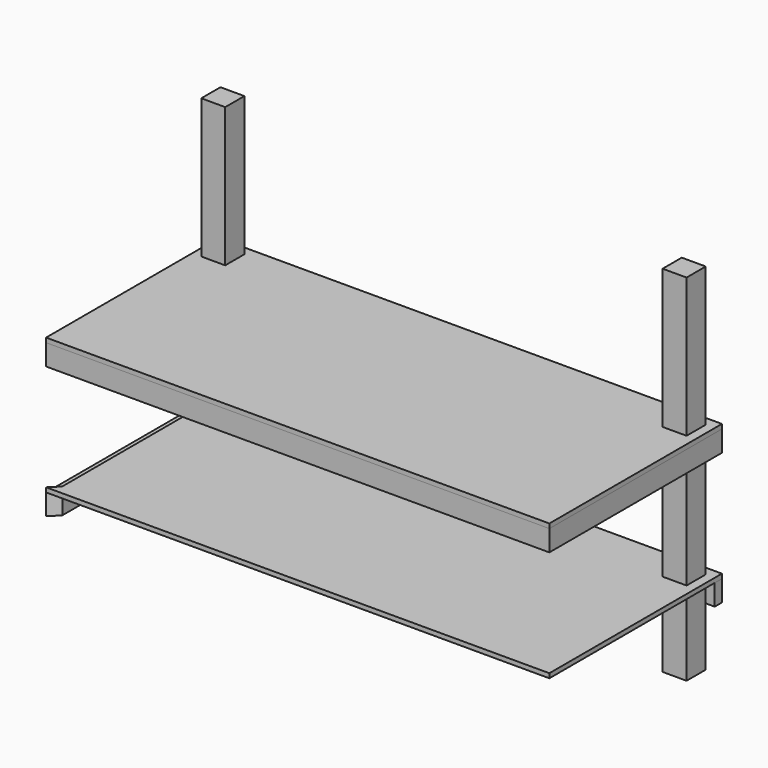
from build123d import *

# Parameters (mm, degrees)
F0_W           = 2133.6
F0_H           = 914.4
F0_W_2         = 101.6
F0_H_2         = 101.6
F1_DEPTH       = 19.05
F2_W           = 2133.6
F2_H           = 88.9
F3_DEPTH       = 38.1
F4_SIZE        = 38.09999
F5_SIZE        = 38.09999
F6_W           = 914.4
F6_H           = 88.9
F7_DEPTH       = 38.1
F8_SIZE        = 38.09999
F9_SIZE        = 38.09999
F10_W          = 2133.6
F10_H          = 88.9
F11_DEPTH      = 38.1
F12_SIZE       = 38.09999
F13_SIZE       = 38.09999
F14_W          = 914.4
F14_H          = 88.9
F15_DEPTH      = 38.1
F16_SIZE       = 38.09999
F17_DEPTH      = 914.4
F17_DEPTH_BACK = 590.55
F18_W          = 914.4
F18_H          = 88.9
F19_DEPTH      = 38.1
F20_SIZE       = 38.09999
F23_DEPTH      = 19.05
F21_W          = 2133.6
F21_H          = 88.9
F24_DEPTH      = 38.1
F25_SIZE       = 38.09999


# Not quite as in the source:
# - a fillet or chamfer is up to 0.001 mm smaller than in the source, because OpenCascade refuses the exact size


with BuildPart() as f1:
    # F0 (on Top) → F1 (new body)
    with BuildSketch(Plane.XY):
        Rectangle(F0_W, F0_H)
        with Locations((-977.9, 368.3)):
            Rectangle(F0_W_2, F0_H_2, mode=Mode.SUBTRACT)
        with Locations((977.9, 368.3)):
            Rectangle(F0_W_2, F0_H_2, mode=Mode.SUBTRACT)
    extrude(amount=-F1_DEPTH)


with BuildPart() as f3:
    # F2 (on face) → F3 (new body)
    with BuildSketch(Plane.XZ.offset(457.2)):
        with Locations((0, -63.5)):
            Rectangle(F2_W, F2_H)
    extrude(amount=-F3_DEPTH)

    # F4 (size 38.1 in the source; OpenCascade refuses exactly that, so slightly less here)
    f4_edges = [f3.edges().sort_by_distance(p)[0] for p in [
        (-1066.8, -419.1, -63.5),
    ]]
    chamfer(f4_edges, length=F4_SIZE)

    # F5 (size 38.1 in the source; OpenCascade refuses exactly that, so slightly less here)
    f5_edges = [f3.edges().sort_by_distance(p)[0] for p in [
        (1066.8, -419.1, -63.5),
    ]]
    chamfer(f5_edges, length=F5_SIZE)


with BuildPart() as f7:
    # F6 (on face) → F7 (new body)
    with BuildSketch(Plane.YZ.offset(1066.8)):
        with Locations((0, -63.5)):
            Rectangle(F6_W, F6_H)
    extrude(amount=-F7_DEPTH)

    # F8 (size 38.1 in the source; OpenCascade refuses exactly that, so slightly less here)
    f8_edges = [f7.edges().sort_by_distance(p)[0] for p in [
        (1028.7, -457.2, -63.5),
    ]]
    chamfer(f8_edges, length=F8_SIZE)

    # F9 (size 38.1 in the source; OpenCascade refuses exactly that, so slightly less here)
    f9_edges = [f7.edges().sort_by_distance(p)[0] for p in [
        (1028.7, 457.2, -63.5),
    ]]
    chamfer(f9_edges, length=F9_SIZE)


with BuildPart() as f11:
    # F10 (on face) → F11 (new body)
    with BuildSketch(Plane(origin=(0, 457.2, 0), x_dir=(-1, 0, 0), z_dir=(0, 1, 0))):
        with Locations((0, -63.5)):
            Rectangle(F10_W, F10_H)
    extrude(amount=-F11_DEPTH)

    # F12 (size 38.1 in the source; OpenCascade refuses exactly that, so slightly less here)
    f12_edges = [f11.edges().sort_by_distance(p)[0] for p in [
        (1066.8, 419.1, -63.5),
    ]]
    chamfer(f12_edges, length=F12_SIZE)

    # F13 (size 38.1 in the source; OpenCascade refuses exactly that, so slightly less here)
    f13_edges = [f11.edges().sort_by_distance(p)[0] for p in [
        (-1066.8, 419.1, -63.5),
    ]]
    chamfer(f13_edges, length=F13_SIZE)


with BuildPart() as f15:
    # F14 (on face) → F15 (new body)
    with BuildSketch(Plane(origin=(-1066.8, 0, 0), x_dir=(0, -1, 0), z_dir=(-1, 0, 0))):
        with Locations((0, -63.5)):
            Rectangle(F14_W, F14_H)
    extrude(amount=-F15_DEPTH)

    # F16 (size 38.1 in the source; OpenCascade refuses exactly that, so slightly less here)
    f16_edges = [f15.edges().sort_by_distance(p)[0] for p in [
        (-1028.7, 457.2, -63.5),
        (-1028.7, -457.2, -63.5),
    ]]
    chamfer(f16_edges, length=F16_SIZE)


with BuildPart() as f17:
    # F0 (on Top) → F17 (new body, two sides)
    with BuildSketch(Plane.XY) as f17_sk:
        with Locations((-977.9, 368.3)):
            Rectangle(F0_W_2, F0_H_2)
    extrude(amount=-F17_DEPTH)
    extrude(f17_sk.sketch, amount=F17_DEPTH_BACK)

    # F18 (on face) → F19 (join)
    with BuildSketch(Plane(origin=(-1066.8, 0, 0), x_dir=(0, -1, 0), z_dir=(-1, 0, 0))):
        with Locations((0, -622.3)):
            Rectangle(F18_W, F18_H)
    extrude(amount=-F19_DEPTH)

    # F20 (size 38.1 in the source; OpenCascade refuses exactly that, so slightly less here)
    f20_edges = [f17.edges().sort_by_distance(p)[0] for p in [
        (-1028.7, -457.2, -622.3),
        (-1028.7, 457.2, -622.3),
    ]]
    chamfer(f20_edges, length=F20_SIZE)


with BuildPart() as f17b:
    # F0 (on Top) → F17, piece 2 (new body, two sides)
    with BuildSketch(Plane.XY) as f17_2_sk:
        with Locations((977.9, 368.3)):
            Rectangle(F0_W_2, F0_H_2)
    extrude(amount=-F17_DEPTH)
    extrude(f17_2_sk.sketch, amount=F17_DEPTH_BACK)


with BuildPart() as f23:
    # F22 (on face) → F23 (new body)
    with BuildSketch(Plane.XY.offset(-577.85)):
        Polygon((1066.8, 457.2), (-1066.8, 457.2), (-1028.7, 419.1), (-927.1, 419.1), (-927.1, 317.5), (-1028.7, 317.5), (-1028.7, -419.1), (-1066.8, -457.2), (1066.8, -457.2), align=None)
    extrude(amount=F23_DEPTH)


with BuildPart() as f24:
    # F21 (on face) → F24 (new body)
    with BuildSketch(Plane(origin=(0, 457.2, 0), x_dir=(-1, 0, 0), z_dir=(0, 1, 0))):
        with Locations((0, -622.3)):
            Rectangle(F21_W, F21_H)
    extrude(amount=-F24_DEPTH)

    # F25 (size 38.1 in the source; OpenCascade refuses exactly that, so slightly less here)
    f25_edges = [f24.edges().sort_by_distance(p)[0] for p in [
        (-1066.8, 419.1, -622.3),
    ]]
    chamfer(f25_edges, length=F25_SIZE)


solid = Compound([f1.part, f3.part, f7.part, f11.part, f15.part, f17.part, f17b.part, f23.part, f24.part])
